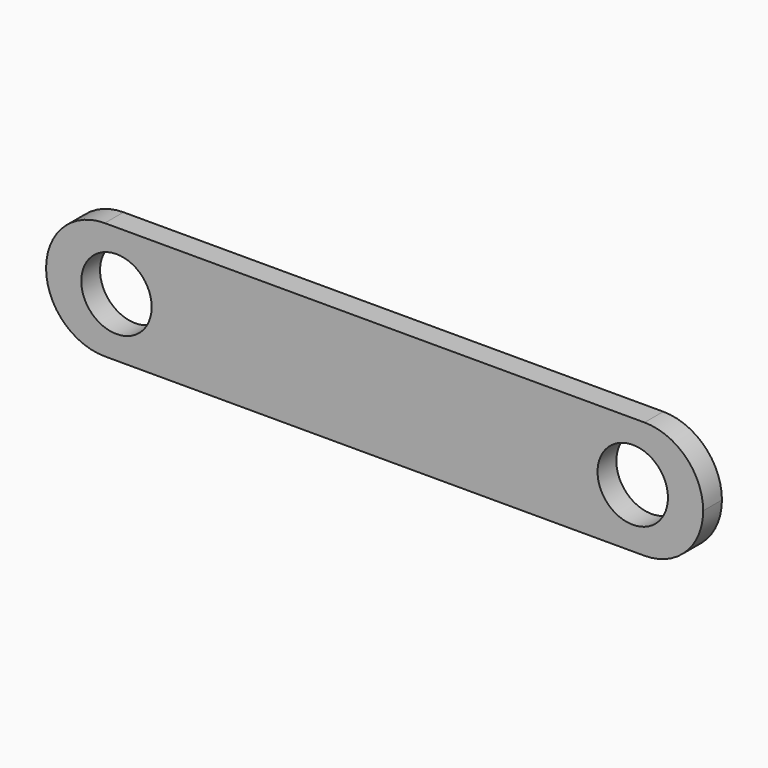
from build123d import *

# Parameters (mm, degrees)
F0_W     = 56
F0_H     = 10
F0_R     = 3
F1_DEPTH = 2
F2_R     = 4.99999


# Not quite as in the source:
# - a fillet or chamfer is up to 0.001 mm smaller than in the source, because OpenCascade refuses the exact size


with BuildPart() as f1:
    # F0 (on Front) → F1 (new body)
    with BuildSketch(Plane.XZ):
        with Locations((-21.8399797827, 0.2435990609)):
            Rectangle(F0_W, F0_H)
        with Locations((-43.8399797827, 0.2435990609)):
            Circle(F0_R, mode=Mode.SUBTRACT)
        with Locations((0.1600202173, 0.2435990609)):
            Circle(F0_R, mode=Mode.SUBTRACT)
    extrude(amount=F1_DEPTH)

    # F2 (radius 5 in the source; OpenCascade refuses exactly that, so slightly less here)
    f2_edges = [f1.edges().sort_by_distance(p)[0] for p in [
        (-49.83998, -1, 5.243599),
        (-49.83998, -1, -4.756401),
        (6.16002, -1, 5.243599),
        (6.16002, -1, -4.756401),
    ]]
    fillet(f2_edges, radius=F2_R)


solid = f1.part
